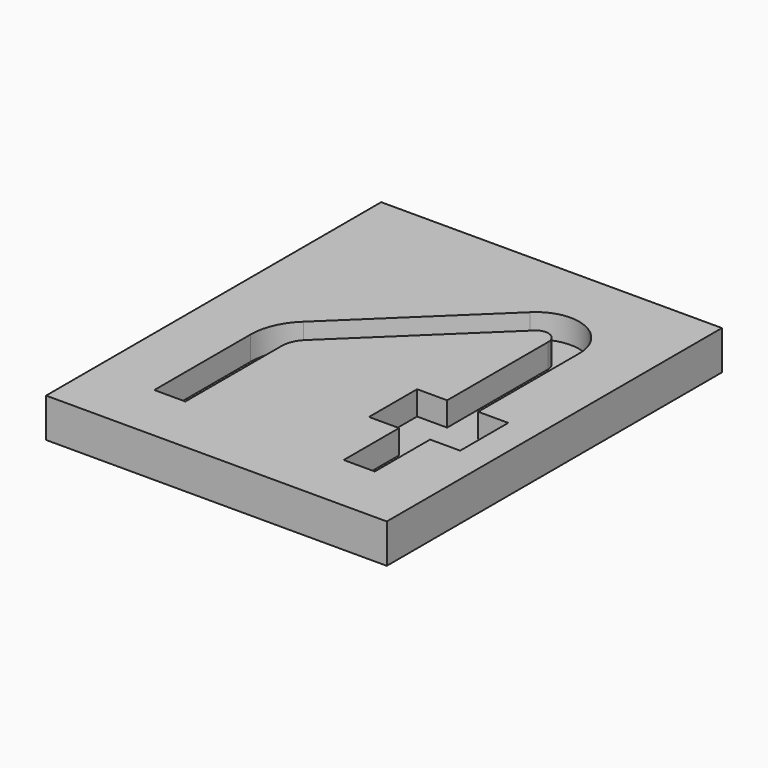
from build123d import *

# Parameters (mm, degrees)
F0_W     = 113.3312
F0_H     = 139.3312
F1_DEPTH = 13
F3_DEPTH = 8


# Not quite as in the source:
# - ends of sketch curves that miss each other by under 0.0002 mm in the source are joined


with BuildPart() as f1:
    # F0 (on Top) → F1 (new body)
    with BuildSketch(Plane.XY):
        Rectangle(F0_W, F0_H)
    extrude(amount=F1_DEPTH)

    # F2 (on face) → F3 (cut)
    with BuildSketch(Plane.XY.offset(13)):
        with BuildLine():
            Line((26.3344, -49.6656), (36.6656, -49.6656))
            Line((36.6656, -49.6656), (36.665598632, -26.6656016949))
            Line((36.665598632, -26.6656016949), (46.6656, -26.6656))
            Line((46.6656, -26.6656), (46.665598632, -6.6656015976))
            Line((46.665598632, -6.6656015976), (36.6656, -6.6656))
            Line((36.6656, -6.6656), (36.6655984, 35.3343984024))
            ThreePointArc((36.6655984, 35.3343984024), (27.823544274, 48.5726978027), (12.2081110977, 45.4754831032))
            Line((12.2081110977, 45.4754831032), (-30.4382024275, 4.5465657527))
            ThreePointArc((-30.4382024275, 4.5465657527), (-35.0404373732, -1.9072796936), (-36.6656, -9.6656))
            Line((-36.6656, -9.6656), (-36.6656, -16.6656))
            Line((-36.6656, -16.6656), (-36.6656, -49.6656))
            Line((-36.6656, -49.6656), (-26.3344000004, -49.6656))
            Line((-26.3344000004, -49.6656), (-26.3344000004, -16.6656))
            Line((-26.3344000004, -16.6656), (-26.3344000004, -9.6656))
            ThreePointArc((-26.3344000004, -9.6656), (-25.6512318575, -6.2260785418), (-23.7054426981, -3.3087285252))
            ThreePointArc((-23.7054426981, -3.3087285252), (-23.7019028512, -3.3051827615), (-23.6983610309, -3.3016389689))
            ThreePointArc((-23.6983610309, -3.3016389689), (-23.566271734, -3.172236103), (-23.4315517652, -3.0455742931))
            Line((-23.4315517652, -3.0455742931), (-11.3959568303, 8.5053390806))
            Line((-11.3959568303, 8.5053390806), (-11.220990014, 8.6732598648))
            Line((-11.220990014, 8.6732598648), (-11.2208270158, 8.6734162989))
            Line((-11.2208270158, 8.6734162989), (9.6364044846, 28.6907129577))
            Line((9.6364044846, 28.6907129577), (9.6666794098, 28.7197686911))
            Line((9.6666794098, 28.7197686911), (19.3337239366, 37.9975147862))
            Line((19.3337239366, 37.9975147862), (19.5059733761, 38.162827624))
            ThreePointArc((19.5059733761, 38.162827624), (23.8651336494, 39.0299159917), (26.334398632, 35.3343983051))
            Line((26.334398632, 35.3343983051), (26.334398632, -6.6656016949))
            Line((26.334398632, -6.6656016949), (16.3344, -6.6656))
            Line((16.3344, -6.6656), (16.334398632, -26.6656016949))
            Line((16.334398632, -26.6656016949), (26.3344, -26.6656))
            Line((26.3344, -26.6656), (26.3344, -49.6656))
        make_face()
        with BuildLine():
            ThreePointArc((-30.988946, 4.018001), (-30.7197680452, 4.2814242377), (-30.4455091202, 4.5395533054))
            Line((-30.4455091202, 4.5395533054), (-30.988946, 4.018001))
        make_face(mode=Mode.SUBTRACT)
        with BuildLine():
            Line((-30.988946, 4.018001), (-30.4455091202, 4.5395533054))
            ThreePointArc((-30.4455091202, 4.5395533054), (-30.7197680452, 4.2814242377), (-30.988946, 4.018001))
        make_face()
        with BuildLine():
            Line((-23.6983610309, -3.3016389689), (-23.4315517652, -3.0455742931))
            ThreePointArc((-23.4315517652, -3.0455742931), (-23.566271734, -3.172236103), (-23.6983610309, -3.3016389689))
        make_face()
        with BuildLine():
            ThreePointArc((-11.2206003272, 8.6733407274), (-11.2207136714, 8.6733785135), (-11.2208270158, 8.6734162989))
            Line((-11.2208270158, 8.6734162989), (-11.220990014, 8.6732598648))
            ThreePointArc((-11.220990014, 8.6732598648), (-11.220876669, 8.6732220799), (-11.2207633243, 8.6731842943))
            Line((-11.2207633243, 8.6731842943), (-11.2206003272, 8.6733407274))
        make_face()
    extrude(amount=-F3_DEPTH, mode=Mode.SUBTRACT)


solid = f1.part
